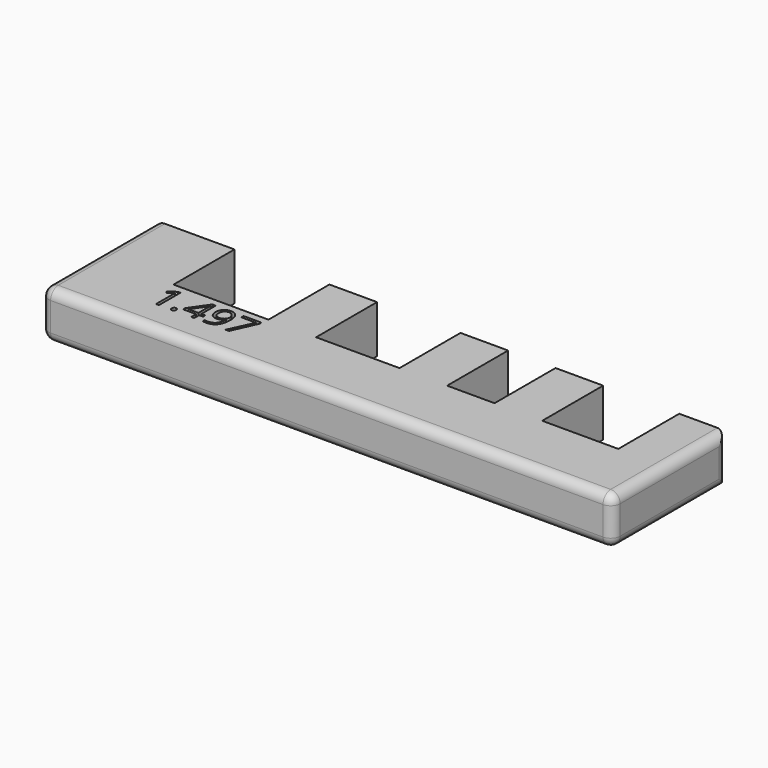
from build123d import *

# Parameters (mm, degrees)
F0_W         = 12.7
F0_H         = 20.32
F1_DEPTH     = 6.35
F2_TEXT_SIZE = 10.0263161585
F3_DEPTH     = 3.175
F4_R         = 2.54


# Not quite as in the source:
# - Text() gives the source's letters only with a copy of the font that has no kerning and outlines rounded to 1/6400 em; it was checked with that copy


with BuildPart() as f1:
    # F0 (on Top) → F1 (new body, symmetric)
    with BuildSketch(Plane.XY):
        Polygon((-76.2, -19.05), (76.2, -19.05), (76.2, 19.05), (63.5, 19.05), (63.5, -1.27), (43.2054, -1.27), (43.2054, 19.05), (30.5054, 19.05), (30.5054, -1.27), (17.8562, -1.27), (17.8562, 19.05), (5.1562, 19.05), (5.1562, -1.27), (-17.0942, -1.27), (-29.7942, -1.27), (-55.118, -1.27), (-55.118, 19.05), (-76.2, 19.05), align=None)
        with Locations((-23.4442, 8.89)):
            Rectangle(F0_W, F0_H)
    extrude(amount=F1_DEPTH, both=True)

    # F2 (on face) → F3 (cut)
    with BuildSketch(Plane.XY.offset(6.35)):
        with Locations((-55.1948715001, -10.3772375733)):
            Text('1.497', F2_TEXT_SIZE, font='Open Sans', text_align=(TextAlign.LEFT, TextAlign.BOTTOM))
    extrude(amount=-F3_DEPTH, mode=Mode.SUBTRACT)

    # F4
    f4_edges = [f1.edges().sort_by_distance(p)[0] for p in [
        (-76.2, 0, 6.35),
        (0, -19.05, 6.35),
        (76.2, 0, 6.35),
        (76.2, 0, -6.35),
        (76.2, -19.05, 0),
        (76.2, 19.05, 0),
        (0, -19.05, -6.35),
        (-76.2, -19.05, 0),
        (-76.2, 0, -6.35),
    ]]
    fillet(f4_edges, radius=F4_R)


solid = f1.part
